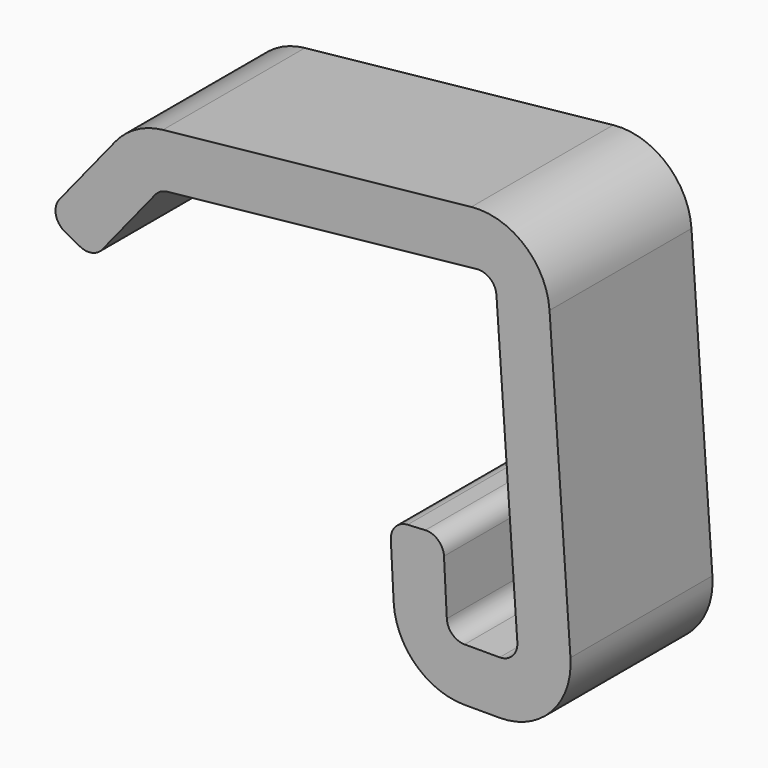
from build123d import *

# Parameters (mm, degrees)
F1_DEPTH = 10
F2_R     = 1
F3_R     = 4


# Not quite as in the source:
# - two fillets or chamfers of one size are made in one step
# - a feature names something its author has since deleted; it is built from what else it names


with BuildPart() as f1:
    # F0 (on Front) → F1 (new body)
    with BuildSketch(Plane.XZ):
        Polygon((30.9209997221, 8.3203603271), (30.6589608257, 13.3203603271), (27.6630722214, 13.1633524584), (28.0741060219, 5.3203603271), (38.1381058522, 5.3203603271), (36.3716140423, 30.5823701452), (13.2265466485, 28.1497255366), (8.2771753479, 22.0377609909), (10.9237883626, 20.6251607112), (14.6997107089, 25.28803648), (33.5956267209, 27.274077282), (34.9209997221, 8.3203603271), align=None)
    extrude(amount=F1_DEPTH)

    # F2
    f2_edges = [f1.edges().sort_by_distance(p)[0] for p in [
        (34.921, -5, 8.32036),
        (30.921, -5, 8.32036),
        (14.699711, -5, 25.288036),
        (8.277175, -5, 22.037761),
        (10.923788, -5, 20.625161),
        (33.595627, -5, 27.274077),
        (30.658961, -5, 13.32036),
        (27.663072, -5, 13.163352),
    ]]
    fillet(f2_edges, radius=F2_R)

    # F3
    f3_edges = [f1.edges().sort_by_distance(p)[0] for p in [
        (38.138106, -5, 5.32036),
        (28.074106, -5, 5.32036),
        (13.226547, -5, 28.149726),
        (36.371614, -5, 30.58237),
    ]]
    fillet(f3_edges, radius=F3_R)


solid = f1.part
